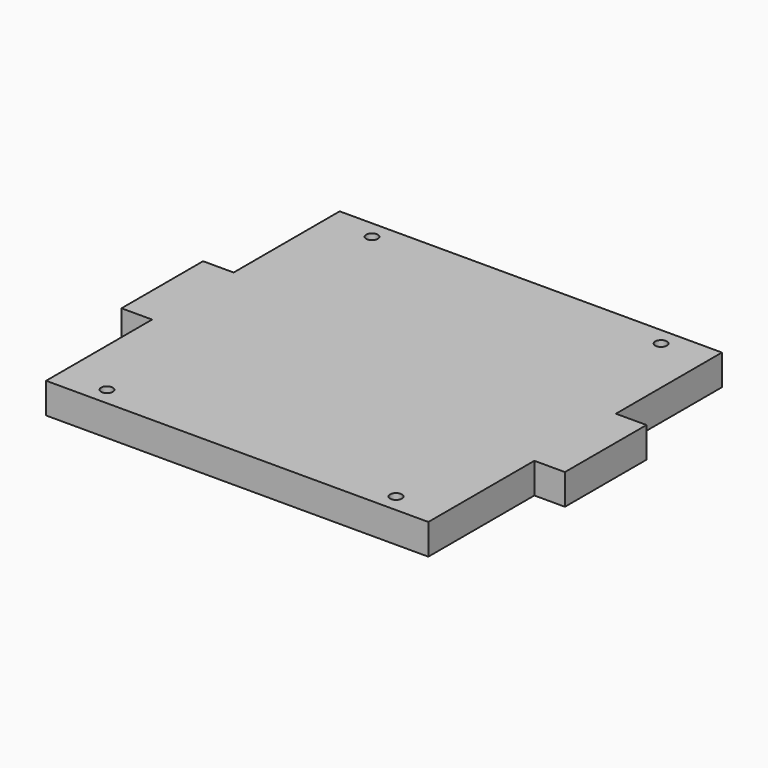
from build123d import *

# Parameters (mm, degrees)
F0_W     = 6
F0_H     = 20
F1_DEPTH = 6
F2_R     = 2.25
F2_R_2   = 1.143
F3_DEPTH = 3
F4_DEPTH = 6


# Not quite as in the source:
# - a feature names something its author has since deleted; it is built from what else it names


with BuildPart() as f1:
    # F0 (on Top) → F1 (new body)
    with BuildSketch(Plane.XY):
        Polygon((-37.5, -36), (37.5, -36), (37.5, -10), (37.5, 10), (37.5, 36), (-37.5, 36), (-37.5, 10), (-37.5, -10), align=None)
        with Locations((40.5, 0)):
            Rectangle(F0_W, F0_H)
        with Locations((-40.5, 0)):
            Rectangle(F0_W, F0_H)
    extrude(amount=F1_DEPTH)

    # F2 (on face) → F3 (cut)
    with BuildSketch(Plane(origin=(0, 0, 0), x_dir=(1, 0, 0), z_dir=(0, 0, -1))):
        with Locations((-28.357, -32.5)):
            Circle(F2_R)
        with Locations((-28.357, -32.5)):
            Circle(F2_R_2, mode=Mode.SUBTRACT)
        with Locations((28.357, -32.5)):
            Circle(F2_R)
        with Locations((28.357, -32.5)):
            Circle(F2_R_2, mode=Mode.SUBTRACT)
        with Locations((-28.357, 32.5)):
            Circle(F2_R)
        with Locations((-28.357, 32.5)):
            Circle(F2_R_2, mode=Mode.SUBTRACT)
        with Locations((28.357, 32.5)):
            Circle(F2_R)
        with Locations((28.357, 32.5)):
            Circle(F2_R_2, mode=Mode.SUBTRACT)
    extrude(amount=-F3_DEPTH, mode=Mode.SUBTRACT)

    # F2 (on face) → F4 (cut, through all)
    with BuildSketch(Plane(origin=(0, 0, 0), x_dir=(1, 0, 0), z_dir=(0, 0, -1))):
        with Locations((-28.357, -32.5)):
            Circle(F2_R_2)
        with Locations((28.357, -32.5)):
            Circle(F2_R_2)
        with Locations((28.357, 32.5)):
            Circle(F2_R_2)
        with Locations((-28.357, 32.5)):
            Circle(F2_R_2)
    extrude(amount=-F4_DEPTH, mode=Mode.SUBTRACT)


solid = f1.part
